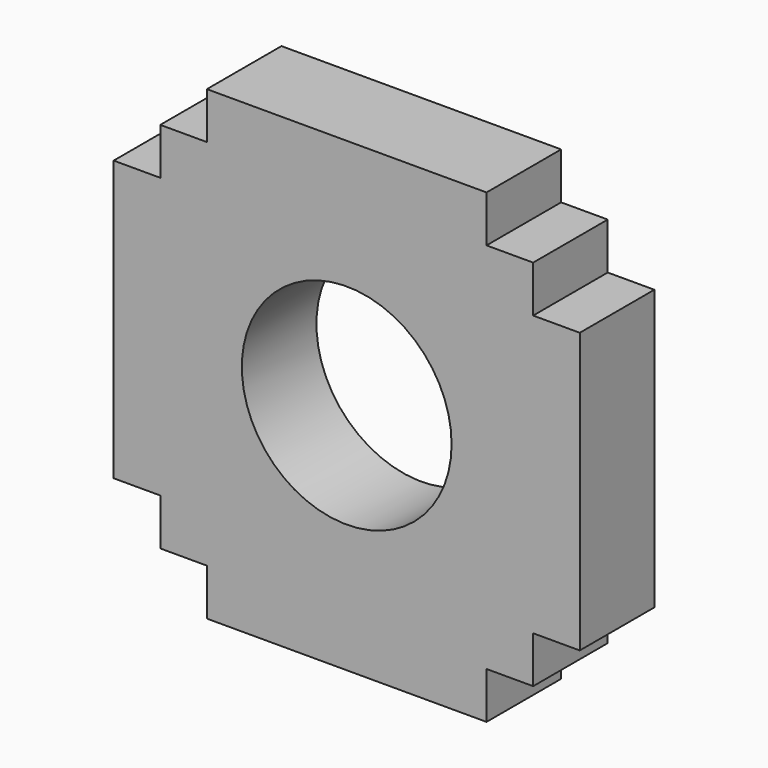
from build123d import *

# Parameters (mm, degrees)
F0_W     = 10
F0_H     = 10
F0_R     = 22.5
F0_W_2   = 0.0176012516
F0_H_2   = 0.0236101449
F0_W_3   = 0.002938509
F0_H_3   = 0.0060267746
F1_DEPTH = 20


with BuildPart() as f1:
    # F0 (on Front) → F1 (new body)
    with BuildSketch(Plane.XZ):
        with Locations((-25, 45)):
            Rectangle(F0_W, F0_H)
        with Locations((-35, 35)):
            Rectangle(F0_W, F0_H)
        Polygon((20, 50), (-20, 50), (-20, 40), (-30, 40), (-30, 30), (-40, 30), (-40, 20), (-50, 20), (-50, -20), (-40, -20), (-40, -30), (-30, -30), (-30, -40), (-20, -40), (-20, -50), (20, -50), (20, -40), (30, -40), (30, -30), (40, -30), (40, -20), (50, -20), (50, 20), (40, 20), (40, 30), (30, 30), (30, 40), (20, 40), align=None)
        Circle(F0_R, mode=Mode.SUBTRACT)
        with Locations((-45, 25)):
            Rectangle(F0_W, F0_H)
        with Locations((25, 45)):
            Rectangle(F0_W, F0_H)
        Polygon((39.9823987484, 40), (30, 40), (30, 30), (40, 30), (40, 39.9763898551), (39.9823987484, 39.9763898551), align=None)
        with Locations((-45, -25)):
            Rectangle(F0_W, F0_H)
        with Locations((39.9911993742, 39.9881949276)):
            Rectangle(F0_W_2, F0_H_2)
        with Locations((45, 25)):
            Rectangle(F0_W, F0_H)
        with Locations((-35, -35)):
            Rectangle(F0_W, F0_H)
        with Locations((-25, -45)):
            Rectangle(F0_W, F0_H)
        with Locations((45, -25)):
            Rectangle(F0_W, F0_H)
        Polygon((40, -39.9939732254), (40, -30), (30, -30), (30, -40), (39.9823987484, -40), (39.997061491, -40), (39.997061491, -39.9939732254), align=None)
        with Locations((25, -45)):
            Rectangle(F0_W, F0_H)
        with Locations((39.9985307455, -39.9969866127)):
            Rectangle(F0_W_3, F0_H_3)
    extrude(amount=F1_DEPTH)


solid = f1.part
